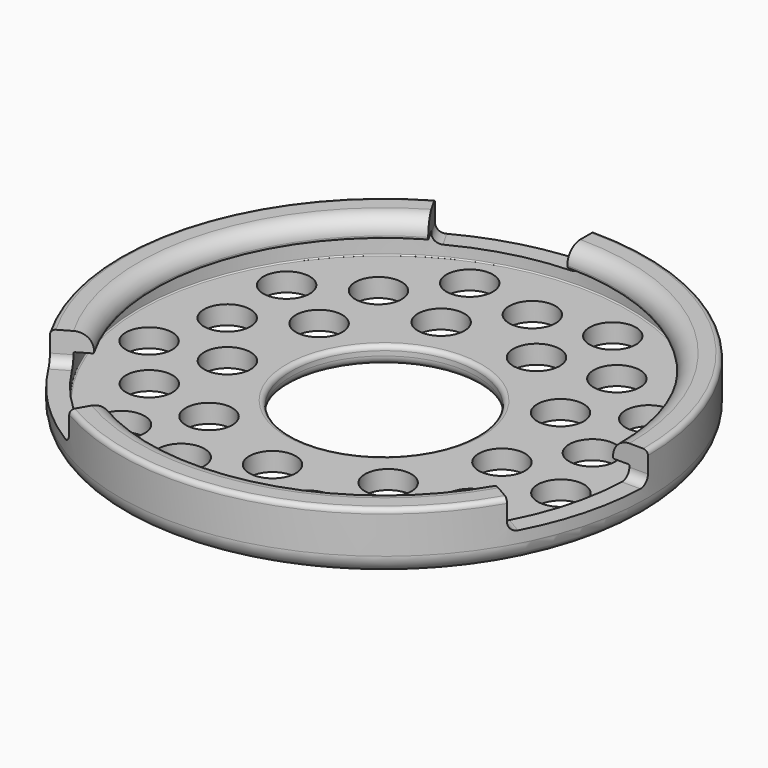
from build123d import *

# Parameters (mm, degrees)
F3_R            = 2.5
F4_DEPTH        = 2
F4_COPIES_COUNT = 9
F7_DEPTH        = 25
F8_R            = 1


# Not quite as in the source:
# - a pattern or mirror of a feature is missing from the dataset's text; its kind, count and spacing are read off the source's solid


with BuildPart() as f2:
    # F0 (on Front) → F2 (revolve)
    with BuildSketch(Plane.XZ):
        with BuildLine():
            ThreePointArc((10, 1), (10.2928932188, 0.2928932188), (11, 0))
            Line((11, 0), (26.4, 0))
            ThreePointArc((26.4, 0), (27.8142135624, 0.5857864376), (28.4, 2))
            Line((28.4, 2), (28.4, 6))
            ThreePointArc((28.4, 6), (28.2535533906, 6.3535533906), (27.9, 6.5))
            Line((27.9, 6.5), (26.4, 6.5))
            ThreePointArc((26.4, 6.5), (25.1625631329, 5.9874368671), (24.65, 4.75))
            Line((24.65, 4.75), (24.65, 4.625))
            ThreePointArc((24.65, 4.625), (24.6866116524, 4.5366116524), (24.775, 4.5))
            Line((24.775, 4.5), (26.275, 4.5))
            ThreePointArc((26.275, 4.5), (26.3633883476, 4.4633883476), (26.4, 4.375))
            Line((26.4, 4.375), (26.4, 2.125))
            ThreePointArc((26.4, 2.125), (26.3633883476, 2.0366116524), (26.275, 2))
            Line((26.275, 2), (10.5, 2))
            ThreePointArc((10.5, 2), (10.1464466094, 1.8535533906), (10, 1.5))
            Line((10, 1.5), (10, 1))
        make_face()
    revolve(axis=Axis((0, 0, 17.7606791258), (0, 0, 1)))

    # F3 (on face) → F4 (cut, through all)
    with BuildSketch(Plane(origin=(0, 0, 0), x_dir=(1, 0, 0), z_dir=(0, 0, -1))):
        with Locations((0, 22.5)):
            Circle(F3_R)
        with Locations((6.8244418925, 18.75)):
            Circle(F3_R)
        with Locations((0, 15)):
            Circle(F3_R)
    f4 = extrude(amount=-F4_DEPTH, mode=Mode.SUBTRACT)

    # F4_copies: F4 ×9 about axis
    f4_copies_axis = Axis((0, 0, 0), (0, 0, 1))
    for i in range(1, F4_COPIES_COUNT):
        add(f4.rotate(f4_copies_axis, i * 360 / F4_COPIES_COUNT), mode=Mode.SUBTRACT)

    # F6 (on offset) → F7 (cut)
    with BuildSketch(Plane.XY.offset(3.25)):
        Polygon((-25, 43.3012701892), (0, 0), (0, 50), align=None)
        Polygon((50, 0), (0, 0), (43.3012701892, -25), align=None)
        Polygon((-25, -43.3012701892), (0, 0), (-43.3012701892, -25), align=None)
    extrude(amount=F7_DEPTH, mode=Mode.SUBTRACT)

    # F8
    f8_edges = [f2.edges().sort_by_distance(p)[0] for p in [
        (0, 27.4, 3.25),
        (-13.7, 23.729096, 3.25),
        (27.4, 0, 3.25),
        (23.729096, -13.7, 3.25),
        (-13.7, -23.729096, 3.25),
        (-23.729096, -13.7, 3.25),
    ]]
    fillet(f8_edges, radius=F8_R)


solid = f2.part
